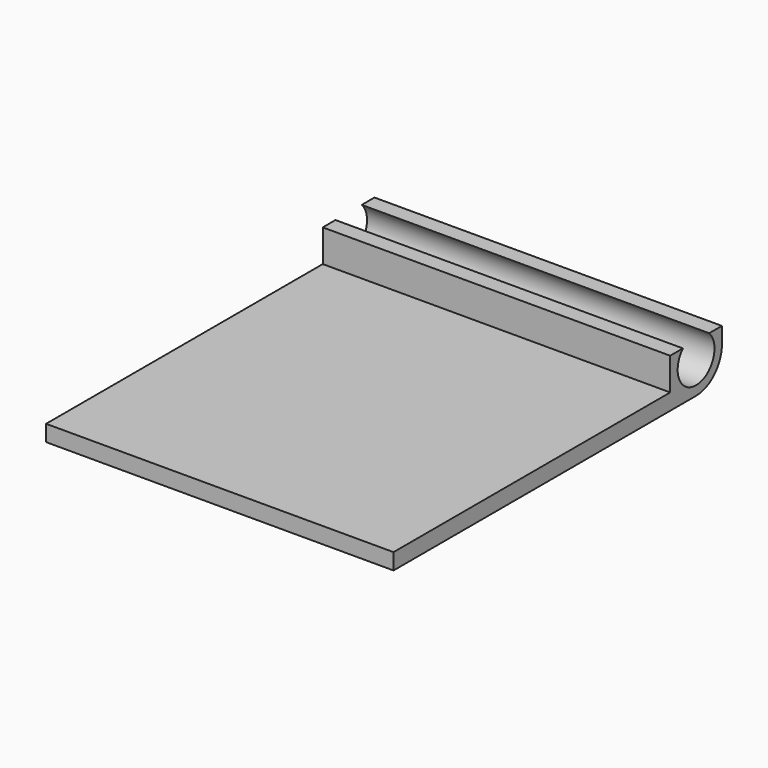
from build123d import *

# Parameters (mm, degrees)
F0_W     = 21.5
F0_H     = 21.4
F1_DEPTH = 1
F0_H_2   = 4
F2_DEPTH = 3
F4_D     = 2.85
F5_R     = 2


# Not quite as in the source:
# - a feature names something its author has since deleted; it is built from what else it names


with BuildPart() as f1:
    # F0 (on Top) → F1 (new body)
    with BuildSketch(Plane.XY):
        Rectangle(F0_W, F0_H)
    extrude(amount=F1_DEPTH)

    # F0 (on Top) → F2 (join)
    with BuildSketch(Plane.XY):
        with Locations((0, 12.7)):
            Rectangle(F0_W, F0_H_2)
    extrude(amount=F2_DEPTH)

    # F4 (through all)
    with Locations(Plane.YZ.offset(10.75)):
        with Locations((12.7, 2)):
            Hole(F4_D / 2)

    # F5
    f5_edges = [f1.edges().sort_by_distance(p)[0] for p in [
        (0, 14.7, 0),
    ]]
    fillet(f5_edges, radius=F5_R)


solid = f1.part
